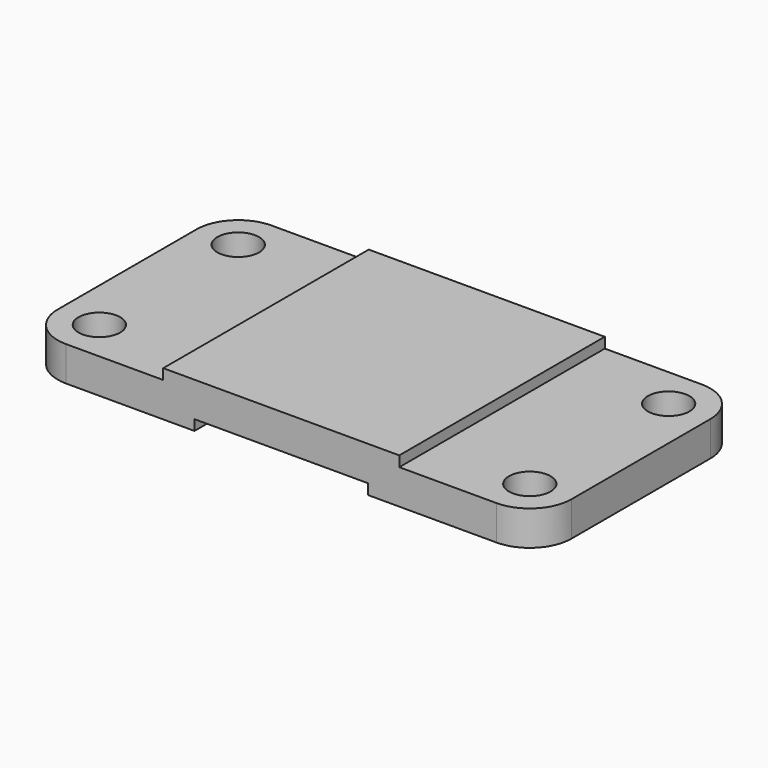
from build123d import *

# Parameters (mm, degrees)
F1_DEPTH = 37
F2_R     = 12
F3_R     = 6
F4_DEPTH = 25


# Not quite as in the source:
# - a pattern or mirror of a feature is missing from the dataset's text; its kind, count and spacing are read off the source's solid


with BuildPart() as f1:
    # F0 (on Front) → F1 (new body, symmetric)
    with BuildSketch(Plane.XZ):
        Polygon((-25, 3), (0, 3), (25, 3), (25, 0), (74, 0), (74, 10), (34, 10), (34, 13), (0, 13), (-34, 13), (-34, 10), (-74, 10), (-74, 0), (-25, 0), align=None)
    extrude(amount=F1_DEPTH, both=True)

    # F2
    f2_edges = [f1.edges().sort_by_distance(p)[0] for p in [
        (74, -37, 5),
        (74, 37, 5),
        (-74, -37, 5),
        (-74, 37, 5),
    ]]
    fillet(f2_edges, radius=F2_R)

    # F3 (on face) → F4 (cut)
    with BuildSketch(Plane.XY.offset(10)):
        with Locations((-62, -25)):
            Circle(F3_R)
    f4 = extrude(amount=-F4_DEPTH, mode=Mode.SUBTRACT)

    # F4_copies: F4 across plane
    add(f4.mirror(Plane.ZX), mode=Mode.SUBTRACT)

    # F4_copies1: F4 across plane
    add(f4.mirror(Plane(origin=(0, 0, 0), x_dir=(-0.3739683355, 0.927441472, 0), z_dir=(0.927441472, 0.3739683355, 0))), mode=Mode.SUBTRACT)

    # F4_copies2: F4 across plane
    add(f4.mirror(Plane(origin=(0, 0, 0), x_dir=(0, 0, 1), z_dir=(1, 0, 0))), mode=Mode.SUBTRACT)


solid = f1.part
